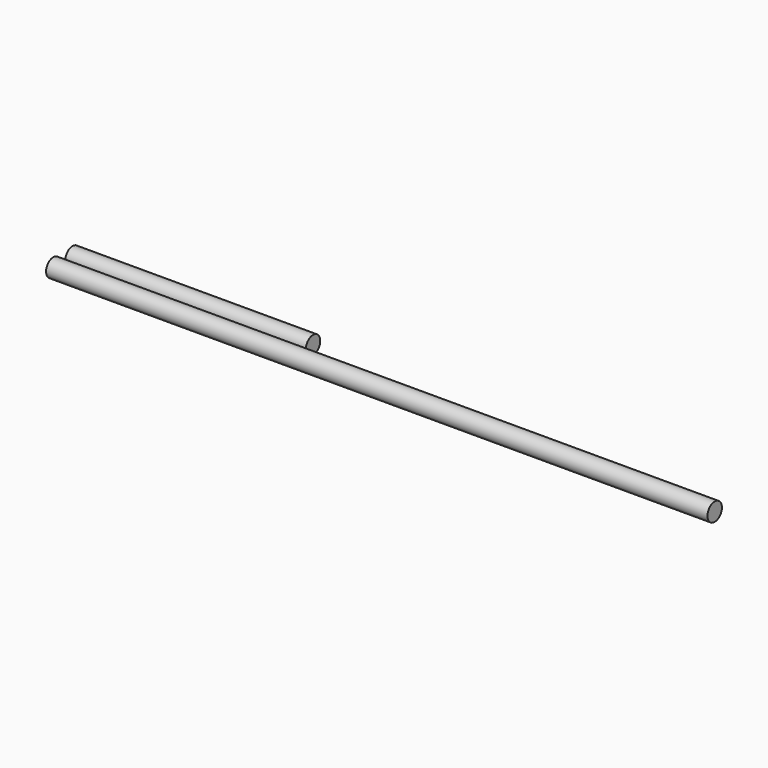
from build123d import *

# Parameters (mm, degrees)
F0_R     = 15
F1_DEPTH = 1100
F2_DEPTH = 400


# Not quite as in the source:
# - a feature names something its author has since deleted; it is built from what else it names


with BuildPart() as f1:
    # F0 (on Right) → F1 (new body)
    with BuildSketch(Plane.YZ):
        Circle(F0_R)
    extrude(amount=F1_DEPTH)


with BuildPart() as f2:
    # F0 (on Right) → F2 (new body)
    with BuildSketch(Plane.YZ):
        with Locations((40, 0)):
            Circle(F0_R)
    extrude(amount=F2_DEPTH)


solid = Compound([f1.part, f2.part])
